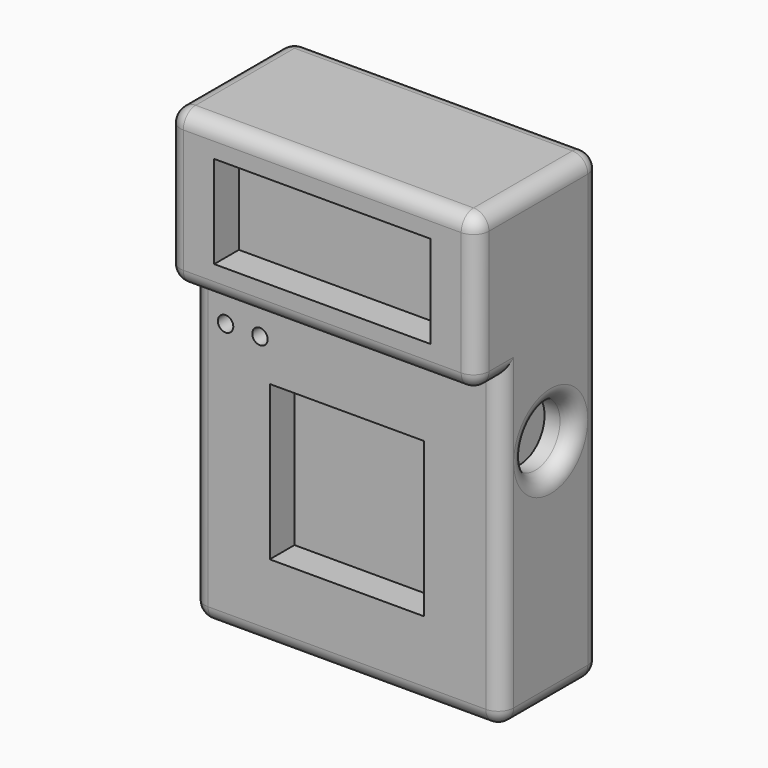
from build123d import *

# Parameters (mm, degrees)
F0_W      = 100
F0_H      = 50
F1_DEPTH  = 50
F3_DEPTH  = 10
F0_H_2    = 100
F4_DEPTH  = 40
F5_R      = 10
F6_DEPTH  = 10
F7_W      = 70
F7_H      = 30
F8_DEPTH  = 10
F9_W      = 30
F9_H      = 10
F10_DEPTH = 10
F11_W     = 50
F11_H     = 50
F12_DEPTH = 10
F13_R     = 4.99999
F14_R     = 2.5
F15_DEPTH = 10


# Not quite as in the source:
# - a fillet or chamfer is up to 0.001 mm smaller than in the source, because OpenCascade refuses the exact size


with BuildPart() as f1:
    # F0 (on Front) → F1 (new body)
    with BuildSketch(Plane.XZ):
        with Locations((0, 50)):
            Rectangle(F0_W, F0_H)
    extrude(amount=F1_DEPTH)

    # F2 (on face) → F3 (cut)
    with BuildSketch(Plane.YZ.offset(50)):
        with BuildLine():
            Line((-35, 25), (-15, 25))
            ThreePointArc((-15, 25), (-25, 35), (-35, 25))
        make_face()
        with BuildLine():
            ThreePointArc((-35, 25), (-25, 15), (-15, 25))
            Line((-15, 25), (-35, 25))
        make_face()
    extrude(amount=-F3_DEPTH, mode=Mode.SUBTRACT)

    # F0 (on Front) → F4 (join)
    with BuildSketch(Plane.XZ):
        with Locations((0, 50)):
            Rectangle(F0_W, F0_H)
        with Locations((0, -25)):
            Rectangle(F0_W, F0_H_2)
    extrude(amount=F4_DEPTH)

    # F5 (on face) → F6 (cut)
    with BuildSketch(Plane.YZ.offset(50)):
        with Locations((-20, 0)):
            Circle(F5_R)
    extrude(amount=-F6_DEPTH, mode=Mode.SUBTRACT)

    # F7 (on face) → F8 (cut)
    with BuildSketch(Plane.XZ.offset(50)):
        with Locations((0, 50)):
            Rectangle(F7_W, F7_H)
    extrude(amount=-F8_DEPTH, mode=Mode.SUBTRACT)

    # F9 (on face) → F10 (cut)
    with BuildSketch(Plane(origin=(0, 0, -75), x_dir=(1, 0, 0), z_dir=(0, 0, -1))):
        with Locations((0, 20)):
            Rectangle(F9_W, F9_H)
    extrude(amount=-F10_DEPTH, mode=Mode.SUBTRACT)

    # F11 (on face) → F12 (cut)
    with BuildSketch(Plane.XZ.offset(40)):
        with Locations((0, -25)):
            Rectangle(F11_W, F11_H)
    extrude(amount=-F12_DEPTH, mode=Mode.SUBTRACT)

    # F13 (radius 5 in the source; OpenCascade refuses exactly that, so slightly less here)
    f13_edges = [f1.edges().sort_by_distance(p)[0] for p in [
        (0, -50, 75),
        (-50, -50, 50),
        (50, -50, 50),
        (0, -50, 25),
        (-50, -40, -25),
        (50, -40, -25),
        (0, -40, -75),
        (0, 0, 75),
        (-50, 0, 0),
        (50, -25, 75),
        (-50, -25, 75),
        (50, 0, 0),
        (50, -20, -75),
        (50, -45, 25),
        (50, -30, 0),
        (0, 0, -75),
        (-50, -20, -75),
        (-50, -45, 25),
    ]]
    fillet(f13_edges, radius=F13_R)

    # F14 (on face) → F15 (cut)
    with BuildSketch(Plane.XZ.offset(40)):
        with Locations((-39.3138879017, 12.5)):
            Circle(F14_R)
        with Locations((-28.179211659, 12.5)):
            Circle(F14_R)
    extrude(amount=-F15_DEPTH, mode=Mode.SUBTRACT)


solid = f1.part
